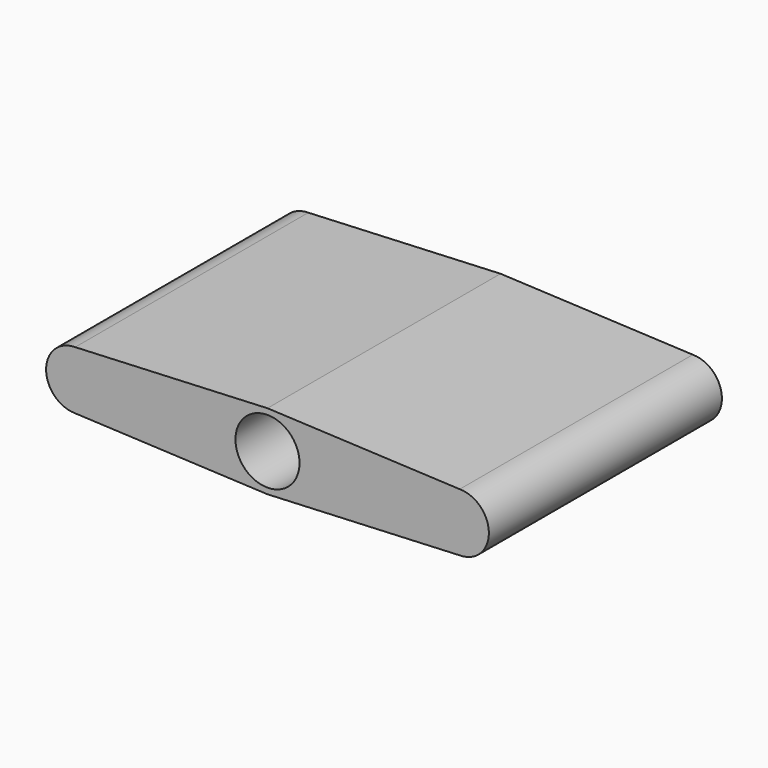
from build123d import *

# Parameters (mm, degrees)
F0_R     = 2.75
F1_DEPTH = 25


# Not quite as in the source:
# - a feature of the source that left no trace in its solid (it failed there, or was rolled back) is left out


with BuildPart() as f1:
    # F0 (on Front) → F1 (new body)
    with BuildSketch(Plane.XZ):
        Polygon((0, 3.25), (-16.5, 2.5), (-16.5, -2.5), (0, -3.25), (16.5, -2.5), (16.5, 2.5), align=None)
        Circle(F0_R, mode=Mode.SUBTRACT)
        with BuildLine():
            Line((-16.5, -2.5), (-16.5, 2.5))
            ThreePointArc((-16.5, 2.5), (-19, 0), (-16.5, -2.5))
        make_face()
        with BuildLine():
            ThreePointArc((16.5, -2.5), (19, 0), (16.5, 2.5))
            Line((16.5, 2.5), (16.5, -2.5))
        make_face()
    extrude(amount=F1_DEPTH)


solid = f1.part
